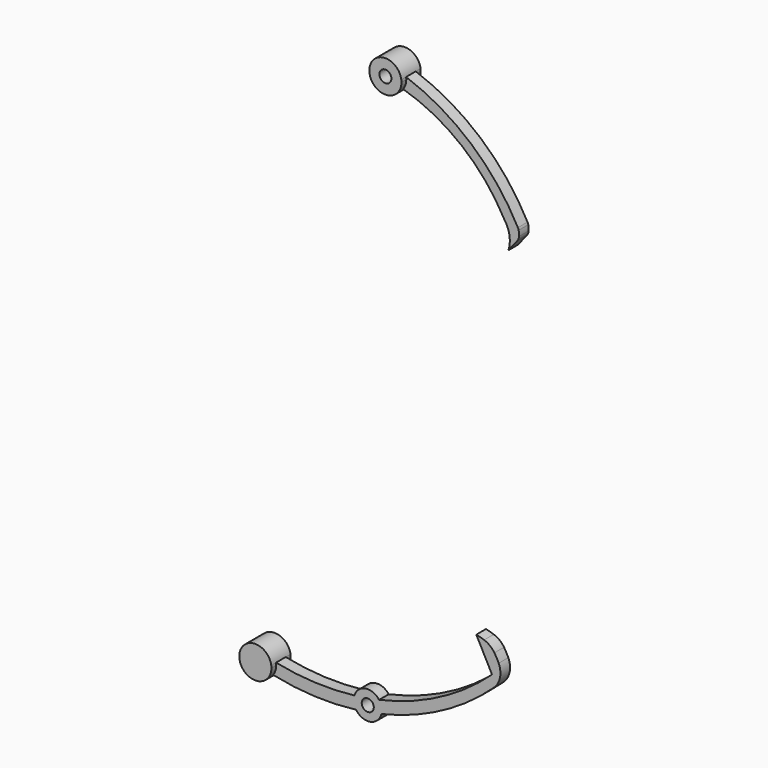
from build123d import *

# Parameters (mm, degrees)
F0_R     = 1.5
F1_DEPTH = 1.5
F0_R_2   = 3
F2_DEPTH = 3
F3_DEPTH = 3
F4_R     = 5
F5_DEPTH = 1.5
F6_DEPTH = 3
F7_R     = 2


with BuildPart() as f1:
    # F0 (on Front) → F1 (new body, symmetric)
    with BuildSketch(Plane.XZ):
        with BuildLine():
            ThreePointArc((-26.34219, -71.276034), (-16.058747, -72.609695), (-5.697339, -72.198498))
            ThreePointArc((-5.697339, -72.198498), (-2.181593, -73.689218), (0.604666, -71.077807))
            ThreePointArc((0.604666, -71.077807), (16.955145, -64.717781), (30.84781, -54.004148))
            ThreePointArc((30.84781, -54.004148), (29.746299, -50.358077), (27.698647, -47.146491))
            ThreePointArc((27.698647, -47.146491), (25.991665, -46.478356), (24.222658, -45.99793))
            Line((24.222658, -45.99793), (28.135919, -53.470021))
            ThreePointArc((28.135919, -53.470021), (15.050222, -62.676034), (0.02157, -68.164727))
            ThreePointArc((0.02157, -68.164727), (-3.377934, -66.79227), (-6.137191, -69.20614))
            ThreePointArc((-6.137191, -69.20614), (-15.913929, -69.559013), (-25.621437, -68.345171))
            ThreePointArc((-25.621437, -68.345171), (-25.589657, -68.634801), (-25.579045, -68.925977))
            ThreePointArc((-25.579045, -68.925977), (-25.774612, -70.161408), (-26.34219, -71.276034))
        make_face()
        with Locations((-2.794387, -70.243281)):
            Circle(F0_R, mode=Mode.SUBTRACT)
    extrude(amount=F1_DEPTH, both=True)

    # F0 (on Front) → F2 (join, symmetric)
    with BuildSketch(Plane.XZ):
        with BuildLine():
            ThreePointArc((-25.621437, -68.345171), (-33.463317, -67.970763), (-26.34219, -71.276034))
            ThreePointArc((-26.34219, -71.276034), (-25.774612, -70.161408), (-25.579045, -68.925977))
            ThreePointArc((-25.579045, -68.925977), (-25.589657, -68.634801), (-25.621437, -68.345171))
        make_face()
        with Locations((-29.579045, -68.925977)):
            Circle(F0_R_2, mode=Mode.SUBTRACT)
    extrude(amount=F2_DEPTH, both=True)

    # F0 (on Front) → F3 (join, symmetric)
    with BuildSketch(Plane.XZ):
        with Locations((-29.579045, -68.925977)):
            Circle(F0_R_2)
    extrude(amount=F3_DEPTH, both=True)

    # F4
    f4_edges = [f1.edges().sort_by_distance(p)[0] for p in [
        (30.84781, 0, -54.004148),
        (27.698647, 0, -47.146491),
    ]]
    fillet(f4_edges, radius=F4_R)


with BuildPart() as f5:
    # F0 (on Front) → F5 (new body, symmetric)
    with BuildSketch(Plane.XZ):
        with BuildLine():
            ThreePointArc((31.199135, 47.250508), (32.483516, 44.164175), (32.220304, 40.831638))
            Line((32.220304, 40.831638), (34.755978, 44.04202))
            ThreePointArc((34.755978, 44.04202), (34.868795, 45.195219), (34.693388, 46.34057))
            ThreePointArc((34.693388, 46.34057), (23.007336, 61.074082), (6.755641, 70.53572))
            ThreePointArc((6.755641, 70.53572), (6.785322, 70.255724), (6.795231, 69.974333))
            ThreePointArc((6.795231, 69.974333), (6.599666, 68.738906), (6.032091, 67.624282))
            ThreePointArc((6.032091, 67.624282), (20.64546, 59.944797), (31.199135, 47.250508))
        make_face()
    extrude(amount=F5_DEPTH, both=True)

    # F0 (on Front) → F6 (join, symmetric)
    with BuildSketch(Plane.XZ):
        with BuildLine():
            ThreePointArc((6.755641, 70.53572), (-1.086687, 70.939067), (6.032091, 67.624282))
            ThreePointArc((6.032091, 67.624282), (6.599666, 68.738906), (6.795231, 69.974333))
            ThreePointArc((6.795231, 69.974333), (6.785322, 70.255724), (6.755641, 70.53572))
        make_face()
        with Locations((2.795231, 69.974333)):
            Circle(F0_R, mode=Mode.SUBTRACT)
    extrude(amount=F6_DEPTH, both=True)

    # F7
    f7_edges = [f5.edges().sort_by_distance(p)[0] for p in [
        (34.693388, 0, 46.34057),
        (34.755978, 0, 44.04202),
        (31.199135, 0, 47.250508),
    ]]
    fillet(f7_edges, radius=F7_R)


solid = Compound([f1.part, f5.part])
